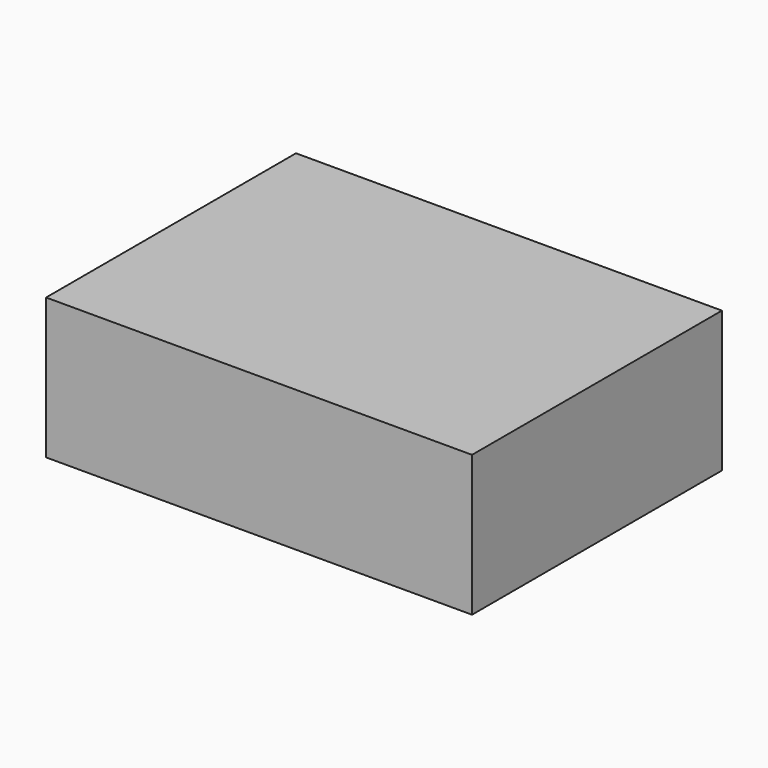
from build123d import *

# Parameters (mm, degrees)
F0_W     = 75.6465587765
F0_H     = 55.4741378874
F1_DEPTH = 25


# Not quite as in the source:
# - a feature names something its author has since deleted; it is built from what else it names


with BuildPart() as f1:
    # F0 (on Top) → F1 (new body)
    with BuildSketch(Plane.XY):
        with Locations((18.7176754698, 8.6314650252)):
            Rectangle(F0_W, F0_H)
    extrude(amount=F1_DEPTH)


solid = f1.part
